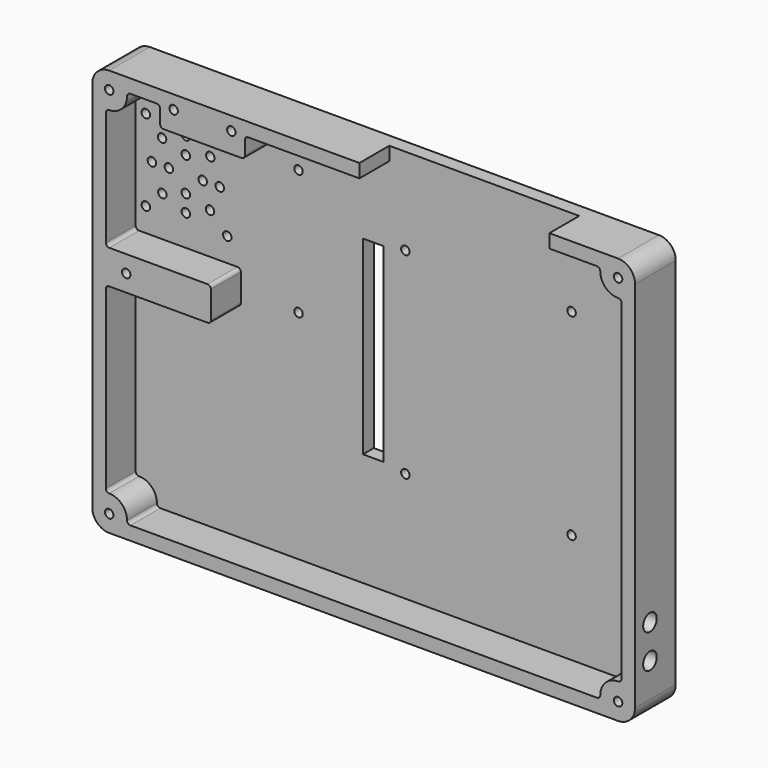
from build123d import *

# Parameters (mm, degrees)
F1_DEPTH  = 15
F2_R      = 1.25
F3_DEPTH  = 25
F4_T      = 4
F5_R      = 1.25
F6_DEPTH  = 25
F7_W      = 56
F7_H      = 4
F8_DEPTH  = 25
F9_W      = 25
F9_H      = 6
F10_DEPTH = 11
F11_R     = 1
F13_D     = 2.5
F13_DEPTH = 10
F13_TIP   = 0.7510757738
F15_D     = 2.5
F15_DEPTH = 10
F15_TIP   = 0.7510757738
F16_R     = 1.25
F17_DEPTH = 11
F18_R     = 1
F20_D     = 2.5
F20_DEPTH = 10
F20_TIP   = 0.7510757738
F21_W     = 6
F21_H     = 56
F22_DEPTH = 25
F24_D     = 5
F24_DEPTH = 100
F24_TIP   = 1.5021515476
F25_R     = 1.25
F26_DEPTH = 5


# Not quite as in the source:
# - a shell that OpenCascade refuses in one call is made with other operations: the cavity is built on its own and cut out


with BuildPart() as f1:
    # F0 (on Front) → F1 (new body)
    with BuildSketch(Plane.XZ):
        with BuildLine():
            Line((-75, -60), (75, -60))
            ThreePointArc((75, -60), (78.5355339059, -58.5355339059), (80, -55))
            Line((80, -55), (80, 55))
            ThreePointArc((80, 55), (78.5355339059, 58.5355339059), (75, 60))
            Line((75, 60), (-75, 60))
            ThreePointArc((-75, 60), (-78.5355339059, 58.5355339059), (-80, 55))
            Line((-80, 55), (-80, -55))
            ThreePointArc((-80, -55), (-78.5355339059, -58.5355339059), (-75, -60))
        make_face()
    extrude(amount=F1_DEPTH)

    # F2 (on Front) → F3 (cut)
    with BuildSketch(Plane.XZ):
        with Locations((-75, 55)):
            Circle(F2_R)
        with Locations((75, 55)):
            Circle(F2_R)
        with Locations((75, -55)):
            Circle(F2_R)
        with Locations((-75, -55)):
            Circle(F2_R)
    extrude(amount=F3_DEPTH, mode=Mode.SUBTRACT)

    # F4: shell of thickness 4, made by hand


with BuildPart() as f4_core1:
    # F4_t2: copy of F1
    add(f1.part)

    # the walls: a layer under each face that stays
    f4_faces = [f4_core1.faces().sort_by_distance(p)[0] for p in [
        (0, -7.5, -60),
        (-78.5355339059, -7.5, -58.5355339059),
        (78.5355339059, -7.5, -58.5355339059),
        (0, 0, 0),
        (-80, -7.5, 0),
        (80, -7.5, 0),
        (-78.5355339059, -7.5, 58.5355339059),
        (78.5355339059, -7.5, 58.5355339059),
        (0, -7.5, 60),
        (-76.25, -7.5, -55),
        (73.75, -7.5, -55),
        (-76.25, -7.5, 55),
        (73.75, -7.5, 55),
    ]]
    thicken(f4_faces, amount=-F4_T, mode=Mode.SUBTRACT)


with BuildPart() as f1_1:
    add(f1.part)

    # what is left inside the walls is the cavity
    f4_cavity = [f4_core1.part.solids().sort_by_distance(p)[0] for p in [
        (0, -4.04, -18.666667),
    ]]
    add(f4_cavity, mode=Mode.SUBTRACT)

    # F5 (on face) → F6 (cut)
    with BuildSketch(Plane.XZ.offset(4)):
        with Locations((3.5, 34.4)):
            Circle(F5_R)
        with Locations((52.5, 34.4)):
            Circle(F5_R)
        with Locations((52.5, -23.6)):
            Circle(F5_R)
        with Locations((3.5, -23.6)):
            Circle(F5_R)
    extrude(amount=-F6_DEPTH, mode=Mode.SUBTRACT)

    # F7 (on face) → F8 (cut)
    with BuildSketch(Plane.XZ.offset(4)):
        with Locations((26.75, 58)):
            Rectangle(F7_W, F7_H)
    extrude(amount=F8_DEPTH, mode=Mode.SUBTRACT)

    # F9 (on face) → F10 (join)
    with BuildSketch(Plane.XZ.offset(4)):
        with Locations((-47.5, 53)):
            Rectangle(F9_W, F9_H)
    extrude(amount=F10_DEPTH)

    # F11
    f11_edges = [f1_1.edges().sort_by_distance(p)[0] for p in [
        (-60, -9.5, 56),
        (-60, -9.5, 50),
        (-35, -9.5, 50),
        (-35, -9.5, 56),
    ]]
    fillet(f11_edges, radius=F11_R)

    # F13
    with Locations(Plane.XZ.offset(15)):
        with Locations((-56, 56), (-39, 56)):
            Hole(F13_D / 2, depth=F13_DEPTH)
            with Locations((0, 0, -(F13_DEPTH + F13_TIP / 2))):  # 118° drill point
                Cone(0, F13_D / 2, F13_TIP, mode=Mode.SUBTRACT)

    # F15
    with Locations(Plane.XZ.offset(4)):
        with Locations((-49, 45), (-73, 45), (-73, 21), (-49, 21)):
            Hole(F15_D / 2, depth=F15_DEPTH)
            with Locations((0, 0, -(F15_DEPTH + F15_TIP / 2))):  # 118° drill point
                Cone(0, F15_D / 2, F15_TIP, mode=Mode.SUBTRACT)

    # F16 (on face) → F17 (join)
    with BuildSketch(Plane.XZ.offset(4)):
        with BuildLine():
            Line((-76, 14), (-76, 4))
            Line((-76, 4), (-46, 4))
            ThreePointArc((-46, 4), (-45.2928932188, 4.2928932188), (-45, 5))
            Line((-45, 5), (-45, 13))
            ThreePointArc((-45, 13), (-45.2928932188, 13.7071067812), (-46, 14))
            Line((-46, 14), (-76, 14))
        make_face()
        with Locations((-70, 9)):
            Circle(F16_R, mode=Mode.SUBTRACT)
    extrude(amount=F17_DEPTH)

    # F18
    f18_edges = [f1_1.edges().sort_by_distance(p)[0] for p in [
        (-76, -9.5, 14),
        (-76, -9.5, 4),
        (-69.846118, -9.5, 56),
        (-76, -9.5, 49.846118),
        (-76, -9.5, -49.846118),
        (-69.846118, -9.5, -56),
        (69.846118, -9.5, -56),
        (76, -9.5, -49.846118),
        (76, -9.5, 49.846118),
        (69.846118, -9.5, 56),
    ]]
    fillet(f18_edges, radius=F18_R)

    # F20
    with Locations(Plane.XZ.offset(4)):
        with Locations((-61.220435021, 43.0927334726), (-61.220435021, 38.0927334726), (-68.2273637709, 40.2273637709), (-71.220435021, 33.0927334726), (-66.220435021, 33.0927334726), (-68.1331846448, 25.8668153552), (-61.220435021, 28.0927334726), (-61.220435021, 23.0927334726), (-53.9945169036, 40.0054830964), (-56.220435021, 33.0927334726), (-54.0858047227, 26.0858047227), (-51.220435021, 33.0927334726)):
            Hole(F20_D / 2, depth=F20_DEPTH)
            with Locations((0, 0, -(F20_DEPTH + F20_TIP / 2))):  # 118° drill point
                Cone(0, F20_D / 2, F20_TIP, mode=Mode.SUBTRACT)

    # F21 (on face) → F22 (cut)
    with BuildSketch(Plane.XZ.offset(4)):
        with Locations((-6, 5.4)):
            Rectangle(F21_W, F21_H)
    extrude(amount=-F22_DEPTH, mode=Mode.SUBTRACT)

    # F24 (one way)
    with BuildSketch(Plane(origin=(0, 0, 0), x_dir=(0, 1, 0), z_dir=(-1, 0, 0))):
        with Locations((-9.5, 35), (-9.5, 45)):
            Circle(F24_D / 2)
    extrude(amount=-F24_DEPTH, mode=Mode.SUBTRACT)
    with Locations(Plane(origin=(0, 0, 0), x_dir=(0, 1, 0), z_dir=(-1, 0, 0))):
        with Locations((-9.5, 35), (-9.5, 45)):
            with Locations((0, 0, -(F24_DEPTH + F24_TIP / 2))):  # 118° drill point
                Cone(0, F24_D / 2, F24_TIP, mode=Mode.SUBTRACT)

    # F25 (on face) → F26 (cut)
    with BuildSketch(Plane.XZ.offset(4)):
        with Locations((-28, 45)):
            Circle(F25_R)
        with Locations((-28, 8)):
            Circle(F25_R)
    extrude(amount=-F26_DEPTH, mode=Mode.SUBTRACT)


solid = f1_1.part
